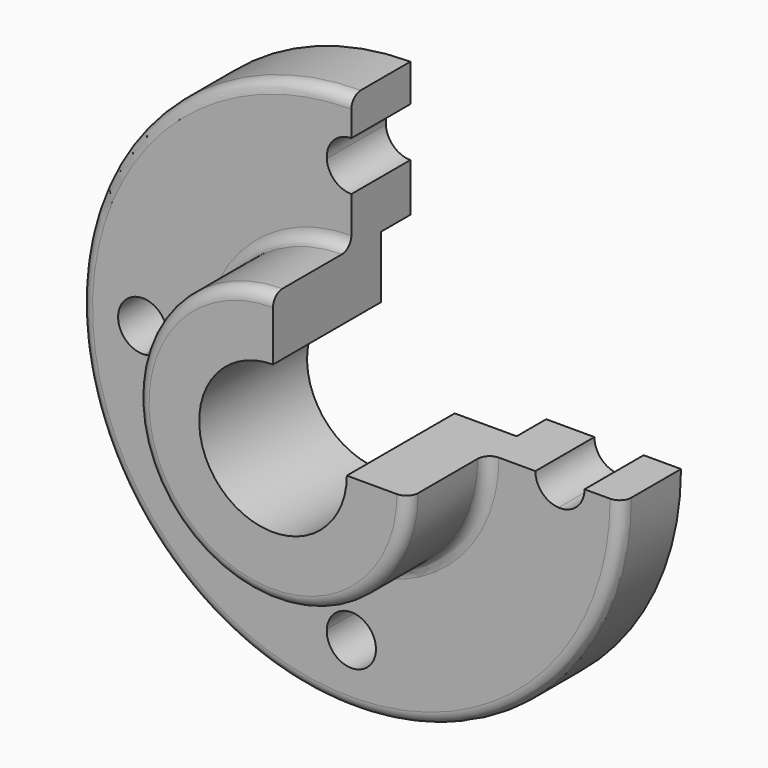
from build123d import *

# Parameters (mm, degrees)
F0_R     = 69.85
F0_R_2   = 35.052
F2_DEPTH = 9.525
F1_R     = 35.052
F1_R_2   = 19.05
F3_DEPTH = 34.798
F4_R     = 3.048
F6_DEPTH = 34.799
F8_DEPTH = 9.526


with BuildPart() as f2:
    # F0 (on Front) → F2 (new body, symmetric)
    with BuildSketch(Plane.XZ):
        Circle(F0_R)
        with BuildLine():
            ThreePointArc((53.47359, 6.338952), (58.203743, 4.620606), (60.198, 0))
            ThreePointArc((60.198, 0), (58.203743, -4.620606), (53.47359, -6.338952))
            ThreePointArc((53.47359, -6.338952), (38.076286, -38.076286), (6.338952, -53.47359))
            ThreePointArc((6.338952, -53.47359), (6.347237, -53.660713), (6.35, -53.848))
            ThreePointArc((6.35, -53.848), (-0.187287, -60.195237), (-6.338952, -53.47359))
            ThreePointArc((-6.338952, -53.47359), (-38.076286, -38.076286), (-53.47359, -6.338952))
            ThreePointArc((-53.47359, -6.338952), (-60.198, 0), (-53.47359, 6.338952))
            ThreePointArc((-53.47359, 6.338952), (-38.076286, 38.076286), (-6.338952, 53.47359))
            ThreePointArc((-6.338952, 53.47359), (-0.187287, 60.195237), (6.35, 53.848))
            ThreePointArc((6.35, 53.848), (6.347237, 53.660713), (6.338952, 53.47359))
            ThreePointArc((6.338952, 53.47359), (38.076286, 38.076286), (53.47359, 6.338952))
        make_face(mode=Mode.SUBTRACT)
        with BuildLine():
            ThreePointArc((53.47359, -6.338952), (47.498, 0), (53.47359, 6.338952))
            ThreePointArc((53.47359, 6.338952), (38.076286, 38.076286), (6.338952, 53.47359))
            ThreePointArc((6.338952, 53.47359), (0, 47.498), (-6.338952, 53.47359))
            ThreePointArc((-6.338952, 53.47359), (-38.076286, 38.076286), (-53.47359, 6.338952))
            ThreePointArc((-53.47359, 6.338952), (-49.227394, 4.355743), (-47.498, 0))
            ThreePointArc((-47.498, 0), (-49.227394, -4.355743), (-53.47359, -6.338952))
            ThreePointArc((-53.47359, -6.338952), (-38.076286, -38.076286), (-6.338952, -53.47359))
            ThreePointArc((-6.338952, -53.47359), (0, -47.498), (6.338952, -53.47359))
            ThreePointArc((6.338952, -53.47359), (38.076286, -38.076286), (53.47359, -6.338952))
        make_face()
        Circle(F0_R_2, mode=Mode.SUBTRACT)
    extrude(amount=F2_DEPTH, both=True)

    # F1 (on Front) → F3 (join)
    with BuildSketch(Plane.XZ):
        Circle(F1_R)
        Circle(F1_R_2, mode=Mode.SUBTRACT)
    extrude(amount=F3_DEPTH)

    # F4
    f4_edges = [f2.edges().sort_by_distance(p)[0] for p in [
        (-35.052, -9.525, 0),
        (-35.052, -34.798, 0),
        (-69.85, -9.525, 0),
    ]]
    fillet(f4_edges, radius=F4_R)

    # F5 (on Front) → F6 (cut, through all)
    with BuildSketch(Plane.XZ):
        Polygon((76.138549, 76.138549), (0, 76.322906), (0, 0), (76.138549, 0), align=None)
    extrude(amount=F6_DEPTH, mode=Mode.SUBTRACT)

    # F7 (on Front) → F8 (cut, through all)
    with BuildSketch(Plane.XZ):
        Polygon((76.691613, 76.322906), (0, 76.138549), (0, 0), (76.691613, 0), align=None)
    extrude(amount=-F8_DEPTH, mode=Mode.SUBTRACT)


solid = f2.part
